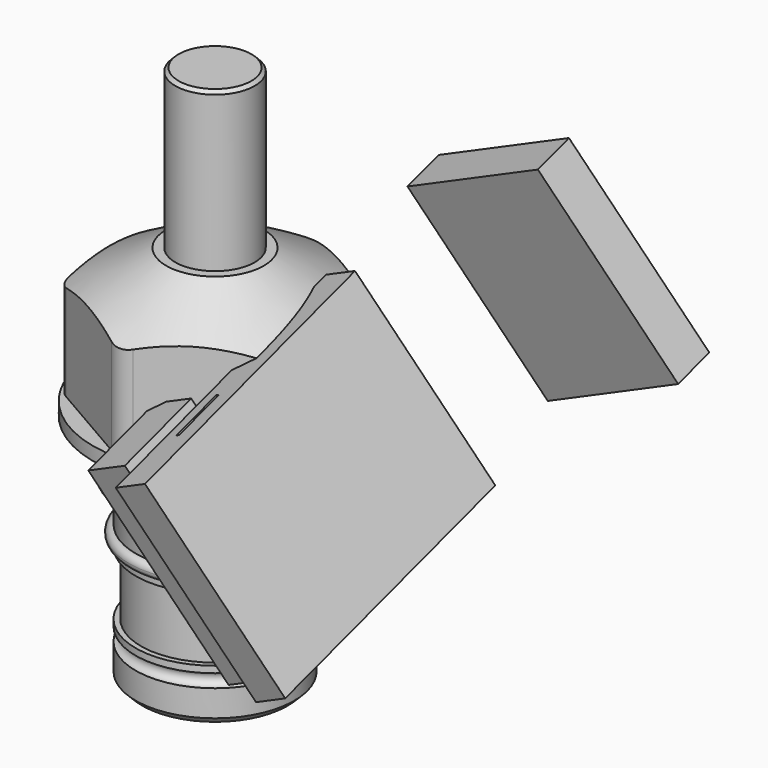
from build123d import *

# Parameters (mm, degrees)
F0_R      = 7.9375
F1_DEPTH  = 35.56
F2_DEPTH  = 3.175
F3_R      = 5.08
F7_SIZE   = 1.5875
F9_DEPTH  = 29.3303937748
F10_W     = 9.525
F10_H     = 37.465
F10_W_2   = 3.175
F10_W_3   = 12.7
F10_H_2   = 22.606
F13_SIZE  = 0.79375
F16_W     = 11.1821069596
F16_H     = 20.8460465074
F16_W_2   = 8.9430306107
F16_H_2   = 65.9904703498
F16_W_3   = 0.8175138473
F16_H_3   = 12.4714046781
F17_DEPTH = 50.8
F16_W_4   = 39.9282462895
F16_H_4   = 9.7671896219


with BuildPart() as f1:
    # F0 (on Top) → F1 (new body)
    with BuildSketch(Plane.XY):
        Polygon((25.4, -14.6646968374), (25.4, 14.6646968374), (0, 29.3293936748), (-25.4, 14.6646968374), (-25.4, -14.6646968374), (0, -29.3293936748), align=None)
        Circle(F0_R, mode=Mode.SUBTRACT)
        Circle(F0_R)
    extrude(amount=F1_DEPTH)

    # F0 (on Top) → F2 (join)
    with BuildSketch(Plane.XY):
        with BuildLine():
            ThreePointArc((-25.4, -14.6646968374), (-14.6646968374, -25.4), (0, -29.3293936748))
            Line((0, -29.3293936748), (-25.4, -14.6646968374))
        make_face()
        with BuildLine():
            ThreePointArc((0, -29.3293936748), (14.6646968374, -25.4), (25.4, -14.6646968374))
            Line((25.4, -14.6646968374), (0, -29.3293936748))
        make_face()
        with BuildLine():
            ThreePointArc((25.4, -14.6646968374), (28.3300188199, -7.5910056644), (29.3293936748, 0))
            ThreePointArc((29.3293936748, 0), (28.3300188199, 7.5910056644), (25.4, 14.6646968374))
            Line((25.4, 14.6646968374), (25.4, -14.6646968374))
        make_face()
        Polygon((25.4, -14.6646968374), (25.4, 14.6646968374), (0, 29.3293936748), (-25.4, 14.6646968374), (-25.4, -14.6646968374), (0, -29.3293936748), align=None)
        Circle(F0_R, mode=Mode.SUBTRACT)
        with BuildLine():
            Line((0, 29.3293936748), (25.4, 14.6646968374))
            ThreePointArc((25.4, 14.6646968374), (14.6646968374, 25.4), (0, 29.3293936748))
        make_face()
        with BuildLine():
            Line((-25.4, 14.6646968374), (0, 29.3293936748))
            ThreePointArc((0, 29.3293936748), (-14.6646968374, 25.4), (-25.4, 14.6646968374))
        make_face()
        with BuildLine():
            Line((-25.4, -14.6646968374), (-25.4, 14.6646968374))
            ThreePointArc((-25.4, 14.6646968374), (-29.3293936748, 0), (-25.4, -14.6646968374))
        make_face()
    extrude(amount=F2_DEPTH)

    # F3 (call 1 of 6: OpenCascade refuses the feature's edges together)
    f3_edges = [f1.edges().sort_by_distance(p)[0] for p in [
        (0, -29.329394, 19.3675),
    ]]
    fillet(f3_edges, radius=F3_R)

    # F3#2 (call 2 of 6)
    f3_2_edges = [f1.edges().sort_by_distance(p)[0] for p in [
        (25.4, -14.664697, 19.3675),
    ]]
    fillet(f3_2_edges, radius=F3_R)

    # F3#3 (call 3 of 6)
    f3_3_edges = [f1.edges().sort_by_distance(p)[0] for p in [
        (25.4, 14.664697, 19.3675),
    ]]
    fillet(f3_3_edges, radius=F3_R)

    # F3#4 (call 4 of 6)
    f3_4_edges = [f1.edges().sort_by_distance(p)[0] for p in [
        (0, 29.329394, 19.3675),
    ]]
    fillet(f3_4_edges, radius=F3_R)

    # F3#5 (call 5 of 6)
    f3_5_edges = [f1.edges().sort_by_distance(p)[0] for p in [
        (-25.4, 14.664697, 19.3675),
    ]]
    fillet(f3_5_edges, radius=F3_R)

    # F3#6 (call 6 of 6)
    f3_6_edges = [f1.edges().sort_by_distance(p)[0] for p in [
        (-25.4, -14.664697, 19.3675),
    ]]
    fillet(f3_6_edges, radius=F3_R)

    # F4 (on Right) → F5 (revolve, cut)
    with BuildSketch(Plane.YZ):
        Polygon((35.3962906179, 35.56), (11.7317574699, 35.56), (35.3962906179, 21.8972754168), align=None)
    revolve(axis=Axis((0, 0, 25.9955581278), (0, 0, -1)), mode=Mode.SUBTRACT)

    # F4 (on Right) → F6 (revolve)
    with BuildSketch(Plane.YZ):
        with BuildLine():
            Line((17.78, -27.686), (0, -27.686))
            Line((0, -27.686), (0, -32.131))
            ThreePointArc((0, -32.131), (2.2450640303, -33.0609359697), (3.175, -35.306))
            ThreePointArc((3.175, -35.306), (2.2450640303, -37.5510640303), (0, -38.481))
            Line((0, -38.481), (0, -42.926))
            Line((0, -42.926), (17.78, -42.926))
            Line((17.78, -42.926), (17.78, -27.686))
        make_face()
        with BuildLine():
            Line((19.05, -12.7), (0, -12.7))
            Line((0, -12.7), (0, -14.2875))
            ThreePointArc((0, -14.2875), (2.2450640303, -15.2174359697), (3.175, -17.4625))
            ThreePointArc((3.175, -17.4625), (2.2450640303, -19.7075640303), (0, -20.6375))
            Line((0, -20.6375), (0, -27.686))
            Line((0, -27.686), (17.78, -27.686))
            Line((17.78, -27.686), (19.05, -27.686))
            Line((19.05, -27.686), (19.05, -26.0985))
            ThreePointArc((19.05, -26.0985), (17.4625, -24.511), (19.05, -22.9235))
            Line((19.05, -22.9235), (19.05, -12.7))
        make_face()
        Polygon((22.225, 0), (0, 0), (0, -12.7), (19.05, -12.7), (22.225, -12.7), align=None)
        with BuildLine():
            Line((19.05, -42.926), (17.78, -42.926))
            Line((17.78, -42.926), (0, -42.926))
            Line((0, -42.926), (0, -55.626))
            Line((0, -55.626), (19.05, -55.626))
            Line((19.05, -55.626), (19.05, -47.6885))
            ThreePointArc((19.05, -47.6885), (17.4625, -46.101), (19.05, -44.5135))
            Line((19.05, -44.5135), (19.05, -42.926))
        make_face()
    revolve(axis=Axis((0, 0, 25.9955581278), (0, 0, -1)))

    # F7
    f7_edges = [f1.edges().sort_by_distance(p)[0] for p in [
        (0, -19.05, -55.626),
    ]]
    chamfer(f7_edges, length=F7_SIZE)


with BuildPart() as f8:
    # F4 (on Right) → F8 (revolve)
    with BuildSketch(Plane.YZ):
        with BuildLine():
            Line((0, -20.6375), (0, -14.2875))
            ThreePointArc((0, -14.2875), (-3.175, -17.4625), (0, -20.6375))
        make_face()
    revolve(axis=Axis((0, 0, 25.9955581278), (0, 0, -1)))


with BuildPart() as f8b:
    # F4 (on Right) → F8, piece 2 (revolve)
    with BuildSketch(Plane.YZ):
        with BuildLine():
            ThreePointArc((20.6375, -24.511), (20.1725320151, -23.3884679849), (19.05, -22.9235))
            Line((19.05, -22.9235), (19.05, -26.0985))
            ThreePointArc((19.05, -26.0985), (20.1725320151, -25.6335320151), (20.6375, -24.511))
        make_face()
        with BuildLine():
            Line((19.05, -26.0985), (19.05, -22.9235))
            ThreePointArc((19.05, -22.9235), (17.4625, -24.511), (19.05, -26.0985))
        make_face()
    revolve(axis=Axis((0, 0, 25.9955581278), (0, 0, -1)))


with BuildPart() as f9_tool:
    # F4 (on Right) → F9 (new body, through all)
    with BuildSketch(Plane.YZ):
        with BuildLine():
            Line((0, -20.6375), (0, -14.2875))
            ThreePointArc((0, -14.2875), (-3.175, -17.4625), (0, -20.6375))
        make_face()
        with BuildLine():
            ThreePointArc((3.175, -17.4625), (2.2450640303, -15.2174359697), (0, -14.2875))
            Line((0, -14.2875), (0, -20.6375))
            ThreePointArc((0, -20.6375), (2.2450640303, -19.7075640303), (3.175, -17.4625))
        make_face()
        with BuildLine():
            Line((0, -38.481), (0, -32.131))
            ThreePointArc((0, -32.131), (-3.175, -35.306), (0, -38.481))
        make_face()
        with BuildLine():
            ThreePointArc((3.175, -35.306), (2.2450640303, -33.0609359697), (0, -32.131))
            Line((0, -32.131), (0, -38.481))
            ThreePointArc((0, -38.481), (2.2450640303, -37.5510640303), (3.175, -35.306))
        make_face()
    extrude(amount=F9_DEPTH)


with BuildPart() as f1_1:
    add(f1.part)

    # F9: cut by f9_tool
    add(f9_tool.part, mode=Mode.SUBTRACT)


with BuildPart() as f8_1:
    add(f8.part)

    # F9: cut by f9_tool
    add(f9_tool.part, mode=Mode.SUBTRACT)


with BuildPart() as f11_tool:
    # F10 (on Right) → F11 (revolve)
    with BuildSketch(Plane.YZ):
        Polygon((9.525, 73.66), (0, 73.66), (0, 15.875), (9.525, 15.875), (9.525, 21.374261314), align=None)
        Polygon((9.525, 21.374261314), (9.525, 15.875), (12.7, 15.875), align=None)
        with Locations((4.7625, -2.8575)):
            Rectangle(F10_W, F10_H)
        with Locations((11.1125, -2.8575)):
            Rectangle(F10_W_2, F10_H)
        with Locations((6.35, -39.243)):
            Rectangle(F10_W_3, F10_H_2)
        Polygon((9.525, -21.59), (0, -21.59), (0, -27.94), (12.7, -27.94), (12.7, -21.59), align=None)
    revolve(axis=Axis((0, 0, 11.557), (0, 0, -1)))


with BuildPart() as f1_2:
    add(f1_1.part)

    # F11: cut by f11_tool
    add(f11_tool.part, mode=Mode.SUBTRACT)

    # F16 (on face) → F17 (join)
    with BuildSketch(Plane(origin=(-7.3290037166, -4.2314022687, 13.7570517399), x_dir=(0.8911228373, -0.133400769, 0.4337099535), z_dir=(0.4537621501, 0.2619796995, -0.8517432407))):
        with Locations((19.2882679044, 29.4184051454)):
            Rectangle(F16_W, F16_H)
        with Locations((33.7742967531, 14.238987118)):
            Rectangle(F16_W_2, F16_H_2)
        with Locations((32.9242492139, 25.2310842308)):
            Rectangle(F16_W_3, F16_H_3, mode=Mode.SUBTRACT)
    extrude(amount=F17_DEPTH)


with BuildPart() as f8_2:
    add(f8_1.part)

    # F11: cut by f11_tool
    add(f11_tool.part, mode=Mode.SUBTRACT)


with BuildPart() as f12:
    # F10 (on Right) → F12 (revolve)
    with BuildSketch(Plane.YZ):
        Polygon((9.525, 73.66), (0, 73.66), (0, 15.875), (9.525, 15.875), (9.525, 21.374261314), align=None)
        with Locations((4.7625, -2.8575)):
            Rectangle(F10_W, F10_H)
        Polygon((9.525, -21.59), (0, -21.59), (0, -27.94), (12.7, -27.94), (12.7, -21.59), align=None)
    revolve(axis=Axis((0, 0, 11.557), (0, 0, -1)))

    # F13
    f13_edges = [f12.edges().sort_by_distance(p)[0] for p in [
        (0, -9.525, 73.66),
    ]]
    chamfer(f13_edges, length=F13_SIZE)


with BuildPart() as f17:
    # F16 (on face) → F17, piece 2 (new body)
    with BuildSketch(Plane(origin=(-7.3290037166, -4.2314022687, 13.7570517399), x_dir=(0.8911228373, -0.133400769, 0.4337099535), z_dir=(0.4537621501, 0.2619796995, -0.8517432407))):
        with Locations((47.3870988935, -51.2249916792)):
            Rectangle(F16_W_4, F16_H_4)
    extrude(amount=F17_DEPTH)


solid = Compound([f8b.part, f1_2.part, f12.part, f17.part])
